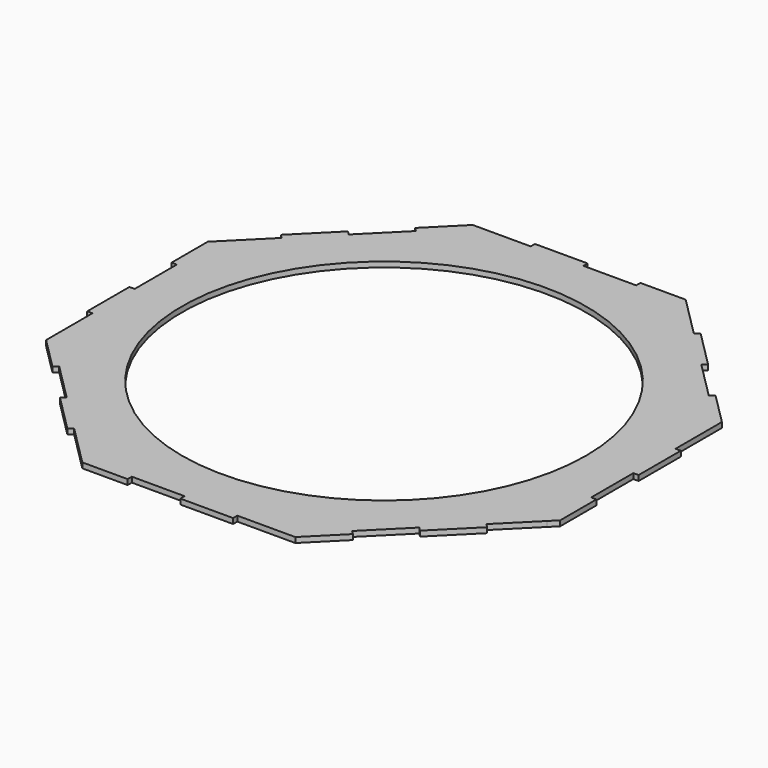
from build123d import *

# Parameters (mm, degrees)
F0_R     = 115
F1_DEPTH = 1.5


with BuildPart() as f1:
    # F0 (on Top) → F1 (new body, symmetric)
    with BuildSketch(Plane.XY):
        Polygon((-59.9971862603, -140.6090075683), (-55.7561938299, -144.85), (-29.9988345097, -144.85), (-29.9988345097, -141.85), (0, -141.85), (0, -144.85), (30, -144.85), (30, -141.85), (56.9988345097, -141.85), (62.9988345097, -141.85), (81.2120379453, -123.6367965644), (79.0907176018, -121.5154762208), (100.3039210374, -100.3022727852), (102.4252413809, -102.4235931288), (123.6384448165, -81.2103896932), (121.517124473, -79.0890693497), (140.609007565, -59.9971862576), (144.85, -55.7561938226), (144.85, -29.9988345097), (141.85, -29.9988345097), (141.85, 0.0011654903), (144.85, 0), (144.85, 30), (141.85, 30), (141.85, 57), (141.85, 62.9988345097), (123.6367965644, 81.2120379453), (121.5154762208, 79.0907176018), (100.3022727852, 100.3039210374), (102.4235931255, 102.4252413776), (81.2103896932, 123.6384448165), (79.0890693497, 121.517124473), (59.9971862576, 140.609007565), (55.7561938226, 144.85), (29.9988345097, 144.85), (29.9988345097, 141.85), (-0.0011654903, 141.85), (0, 144.85), (-30, 144.85), (-30, 141.85), (-57, 141.85), (-62.9988345097, 141.85), (-81.2120379453, 123.6367965644), (-79.0907176018, 121.5154762208), (-100.3039210374, 100.3022727852), (-102.4252413776, 102.4235931255), (-123.6384448165, 81.2103896932), (-121.5171244733, 79.0890693493), (-140.6090075683, 59.9971862603), (-144.85, 55.7561938286), (-144.85, 29.9988345097), (-141.85, 29.9988345097), (-141.85, -0.0011654903), (-144.85, 0), (-144.85, -30), (-141.85, -30), (-141.85, -57), (-141.85, -62.9988345097), (-123.6367965644, -81.2120379453), (-121.5154762208, -79.0907176018), (-100.3022727852, -100.3039210374), (-102.4235931255, -102.4252413776), (-81.2103896932, -123.6384448165), (-79.0890693493, -121.5171244733), align=None)
        Circle(F0_R, mode=Mode.SUBTRACT)
    extrude(amount=F1_DEPTH, both=True)


solid = f1.part
